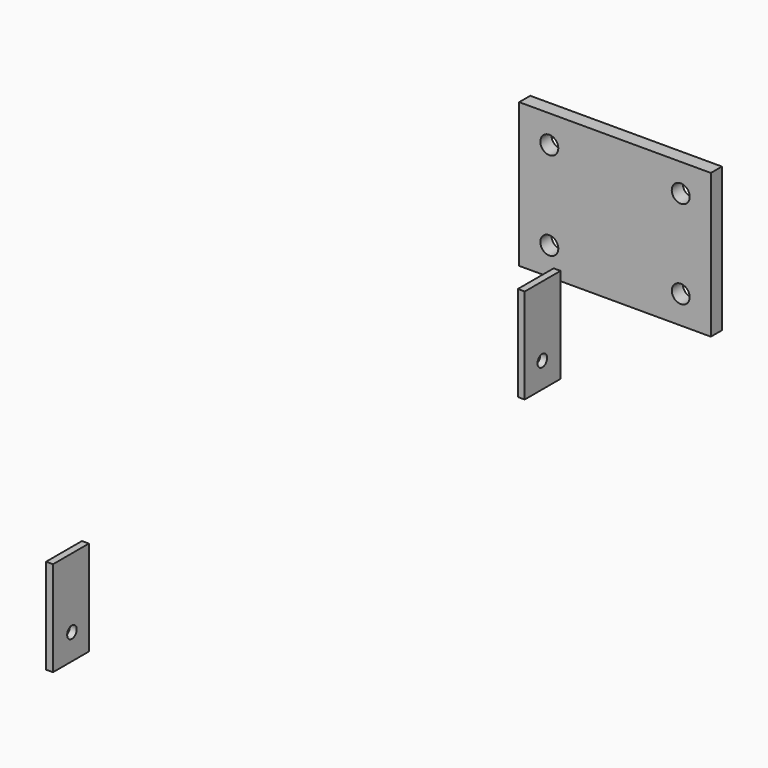
from build123d import *

# Parameters (mm, degrees)
F1_DEPTH  = 2.54
F3_D      = 6.6
F7_W      = 16.4503324777
F7_H      = 34.9378818646
F8_DEPTH  = 1.27
F10_D     = 4.4
F11_W     = 16.4503324777
F11_H     = 34.9378818646
F12_DEPTH = 1.27
F14_D     = 4.4


# Not quite as in the source:
# - the program builds the solid bodies; features that only make, move or delete a surface that nothing else refers to are left out


with BuildPart() as f1:
    # F0 (on Front) → F1 (new body, symmetric)
    with BuildSketch(Plane.XZ):
        Polygon((-25.0618057636, 18.8499050002), (-35.2113864935, 26.4837776091), (-35.2113864935, -26.4837776091), (0, 0), align=None)
        Polygon((35.2113864935, 26.4837776091), (-35.2113864935, 26.4837776091), (-25.0618057636, 18.8499050002), (0, 0), align=None)
        Polygon((35.2113864935, -26.4837776091), (35.2113864935, 26.4837776091), (0, 0), align=None)
        Polygon((0, 0), (-35.2113864935, -26.4837776091), (35.2113864935, -26.4837776091), align=None)
    extrude(amount=F1_DEPTH, both=True)

    # F3 (through all)
    with Locations(Plane.XZ.offset(2.54)):
        with Locations((-24.1408664733, 16.2348244339), (24.1408664733, 16.2348244339), (24.1408664733, -16.2348244339), (-24.1408664733, -16.2348244339)):
            Hole(F3_D / 2)


with BuildPart() as f8:
    # F7 (on Right) → F8 (new body, symmetric)
    with BuildSketch(Plane.YZ):
        with Locations((-37.3634537682, -22.8809299879)):
            Rectangle(F7_W, F7_H)
    extrude(amount=F8_DEPTH, both=True)

    # F10 (through all)
    with Locations(Plane(origin=(-1.27, 0, 0), x_dir=(0, -1, 0), z_dir=(-1, 0, 0))):
        with Locations((37.5186465681, -31.0383625329)):
            Hole(F10_D / 2)


with BuildPart() as f12:
    # F11 (on Right) → F12 (new body, symmetric)
    with BuildSketch(Plane.YZ):
        with Locations((-254.0175085887, -23.0186316185)):
            Rectangle(F11_W, F11_H)
    extrude(amount=F12_DEPTH, both=True)

    # F14 (through all)
    with Locations(Plane(origin=(-1.27, 0, 0), x_dir=(0, -1, 0), z_dir=(-1, 0, 0))):
        with Locations((253.5456418991, -31.0383625329)):
            Hole(F14_D / 2)


solid = Compound([f1.part, f8.part, f12.part])
